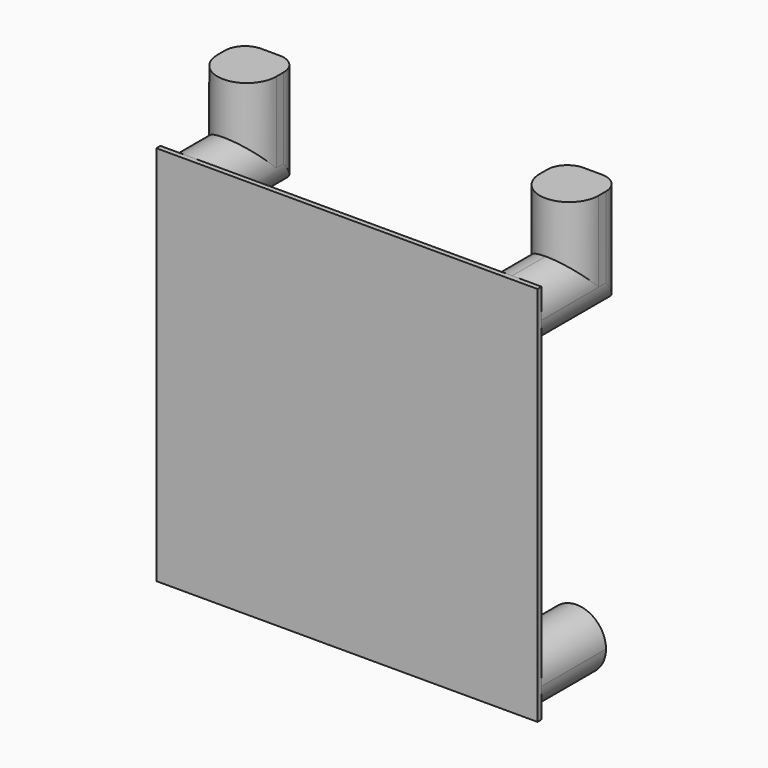
from build123d import *

# Parameters (mm, degrees)
F1_DEPTH    = 0.4
F2_DEPTH    = 6.35
F4_DEPTH    = 7.9375
F6_DEPTH    = 6.35
F7_T1_DEPTH = 14.2875


# Not quite as in the source:
# - a fillet or chamfer that OpenCascade refuses, or shapes differently, is made with other operations: its cross-section is extruded or revolved along the edge and cut away or added
# - a pattern or mirror of a feature is missing from the dataset's text; its kind, count and spacing are read off the source's solid


with BuildPart() as f1:
    # F0 (on Front) → F1 (new body)
    with BuildSketch(Plane.XZ):
        with BuildLine():
            ThreePointArc((-12.7, 15.01775), (-11.0611032579, 14.3388967421), (-10.38225, 12.7))
            ThreePointArc((-10.38225, 12.7), (-12.7, 10.38225), (-15.01775, 12.7))
            Line((-15.01775, 12.7), (-15.01775, -12.7000000336))
            ThreePointArc((-15.01775, -12.7000000336), (-12.7000000168, -10.38225), (-10.38225, -12.7))
            ThreePointArc((-10.38225, -12.7), (-11.0611032579, -14.3388967421), (-12.7, -15.01775))
            Line((-12.7, -15.01775), (12.7, -15.01775))
            ThreePointArc((12.7, -15.01775), (11.0611032579, -11.0611032579), (15.01775, -12.7))
            Line((15.01775, -12.7), (15.01775, 12.7))
            ThreePointArc((15.01775, 12.7), (11.0611032579, 11.0611032579), (12.7, 15.01775))
            Line((12.7, 15.01775), (-12.7, 15.01775))
        make_face()
        with BuildLine():
            ThreePointArc((-10.38225, -12.7), (-12.7000000168, -10.38225), (-15.01775, -12.7000000336))
            ThreePointArc((-15.01775, -12.7000000336), (-14.3388967302, -14.338896754), (-12.7, -15.01775))
            ThreePointArc((-12.7, -15.01775), (-11.0611032579, -14.3388967421), (-10.38225, -12.7))
        make_face()
        with BuildLine():
            ThreePointArc((-15.01775, 12.7), (-12.7, 10.38225), (-10.38225, 12.7))
            ThreePointArc((-10.38225, 12.7), (-11.0611032579, 14.3388967421), (-12.7, 15.01775))
            ThreePointArc((-12.7, 15.01775), (-14.3388967421, 14.3388967421), (-15.01775, 12.7))
        make_face()
        with BuildLine():
            ThreePointArc((15.01775, 12.7), (14.3388967421, 14.3388967421), (12.7, 15.01775))
            ThreePointArc((12.7, 15.01775), (11.0611032579, 11.0611032579), (15.01775, 12.7))
        make_face()
        with BuildLine():
            ThreePointArc((12.7, -15.01775), (14.3388967421, -14.3388967421), (15.01775, -12.7))
            ThreePointArc((15.01775, -12.7), (11.0611032579, -11.0611032579), (12.7, -15.01775))
        make_face()
        with BuildLine():
            ThreePointArc((-15.01775, 12.7), (-14.3388967421, 14.3388967421), (-12.7, 15.01775))
            Line((-12.7, 15.01775), (-15.01775, 15.01775))
            Line((-15.01775, 15.01775), (-15.01775, 12.7))
        make_face()
        with BuildLine():
            Line((15.01775, 15.01775), (12.7, 15.01775))
            ThreePointArc((12.7, 15.01775), (14.3388967421, 14.3388967421), (15.01775, 12.7))
            Line((15.01775, 12.7), (15.01775, 15.01775))
        make_face()
        with BuildLine():
            Line((15.01775, -15.01775), (15.01775, -12.7))
            ThreePointArc((15.01775, -12.7), (14.3388967421, -14.3388967421), (12.7, -15.01775))
            Line((12.7, -15.01775), (15.01775, -15.01775))
        make_face()
        with BuildLine():
            ThreePointArc((-12.7, -15.01775), (-14.3388967302, -14.338896754), (-15.01775, -12.7000000336))
            Line((-15.01775, -12.7000000336), (-15.01775, -15.01775))
            Line((-15.01775, -15.01775), (-12.7, -15.01775))
        make_face()
    extrude(amount=F1_DEPTH)

    # F0 (on Front) → F2 (join)
    with BuildSketch(Plane.XZ):
        with BuildLine():
            ThreePointArc((-15.01775, 12.7), (-12.7, 10.38225), (-10.38225, 12.7))
            ThreePointArc((-10.38225, 12.7), (-11.0611032579, 14.3388967421), (-12.7, 15.01775))
            ThreePointArc((-12.7, 15.01775), (-14.3388967421, 14.3388967421), (-15.01775, 12.7))
        make_face()
        with BuildLine():
            ThreePointArc((-10.38225, -12.7), (-12.7000000168, -10.38225), (-15.01775, -12.7000000336))
            ThreePointArc((-15.01775, -12.7000000336), (-14.3388967302, -14.338896754), (-12.7, -15.01775))
            ThreePointArc((-12.7, -15.01775), (-11.0611032579, -14.3388967421), (-10.38225, -12.7))
        make_face()
        with BuildLine():
            ThreePointArc((12.7, -15.01775), (14.3388967421, -14.3388967421), (15.01775, -12.7))
            ThreePointArc((15.01775, -12.7), (11.0611032579, -11.0611032579), (12.7, -15.01775))
        make_face()
    extrude(amount=-F2_DEPTH)

    # F0 (on Front) → F4 (join)
    with BuildSketch(Plane.XZ):
        with BuildLine():
            ThreePointArc((-15.01775, 12.7), (-12.7, 10.38225), (-10.38225, 12.7))
            ThreePointArc((-10.38225, 12.7), (-11.0611032579, 14.3388967421), (-12.7, 15.01775))
            ThreePointArc((-12.7, 15.01775), (-14.3388967421, 14.3388967421), (-15.01775, 12.7))
        make_face()
        with BuildLine():
            ThreePointArc((15.01775, 12.7), (14.3388967421, 14.3388967421), (12.7, 15.01775))
            ThreePointArc((12.7, 15.01775), (11.0611032579, 11.0611032579), (15.01775, 12.7))
        make_face()
    extrude(amount=-F4_DEPTH)

    # F5 (on plane+point) → F6 (join)
    with BuildSketch(Plane.XY.offset(12.7)):
        with BuildLine():
            Line((15.01775, 5.61975), (15.01775, 7.9375))
            Line((15.01775, 7.9375), (10.38225, 7.9375))
            Line((10.38225, 7.9375), (10.38225, 5.61975))
            ThreePointArc((10.38225, 5.61975), (12.7, 3.302), (15.01775, 5.61975))
        make_face()
    f6 = extrude(amount=F6_DEPTH)

    # F6_copies: F6 across plane
    add(f6.mirror(Plane(origin=(0, 0, 0), x_dir=(0, 0, -1), z_dir=(-1, 0, 0))))

    # F7: fillet of radius 1.5875 on 4 edges, made by hand

    # F7_s2 → F7_t1 (cut)
    with BuildSketch(Plane.XY.offset(8.73125)):
        with BuildLine():
            ThreePointArc((15.01775, 6.35), (14.5527820151, 7.4725320151), (13.43025, 7.9375))
            Line((13.43025, 7.9375), (15.01775, 7.9375))
            Line((15.01775, 7.9375), (15.01775, 6.35))
        make_face()
        with BuildLine():
            ThreePointArc((11.96975, 7.9375), (10.8472179849, 7.4725320151), (10.38225, 6.35))
            Line((10.38225, 6.35), (10.38225, 7.9375))
            Line((10.38225, 7.9375), (11.96975, 7.9375))
        make_face()
        with BuildLine():
            ThreePointArc((-10.38225, 6.35), (-10.8472179849, 7.4725320151), (-11.96975, 7.9375))
            Line((-11.96975, 7.9375), (-10.38225, 7.9375))
            Line((-10.38225, 7.9375), (-10.38225, 6.35))
        make_face()
        with BuildLine():
            ThreePointArc((-13.43025, 7.9375), (-14.5527820151, 7.4725320151), (-15.01775, 6.35))
            Line((-15.01775, 6.35), (-15.01775, 7.9375))
            Line((-15.01775, 7.9375), (-13.43025, 7.9375))
        make_face()
    extrude(amount=F7_T1_DEPTH, mode=Mode.SUBTRACT)


solid = f1.part
